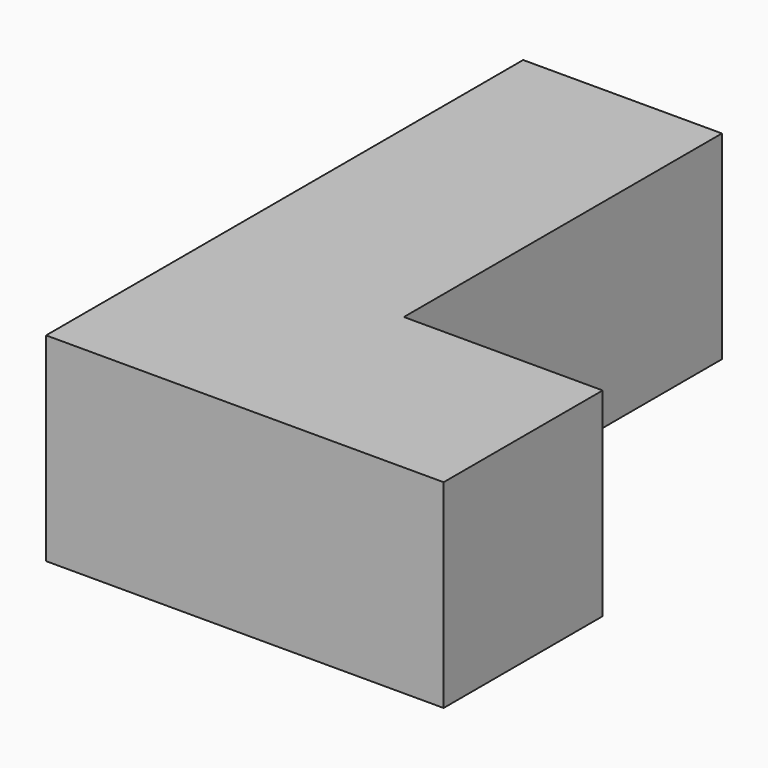
from build123d import *

# Parameters (mm, degrees)
F1_W     = 127
F1_H     = 127
F2_DEPTH = 190.5
F3_W     = 127
F3_H     = 127
F4_DEPTH = 127


# Not quite as in the source:
# - a variable given as a bare number and used for a length is read in inches; the dataset says mm whatever the document's units were


with BuildPart() as f2:
    # F1 (on Front) → F2 (new body, symmetric)
    with BuildSketch(Plane.XZ):
        Rectangle(F1_W, F1_H)
    extrude(amount=F2_DEPTH, both=True)

    # F3 (on face) → F4 (join)
    with BuildSketch(Plane.YZ.offset(63.5)):
        with Locations((-127, 0)):
            Rectangle(F3_W, F3_H)
    extrude(amount=F4_DEPTH)


solid = f2.part
